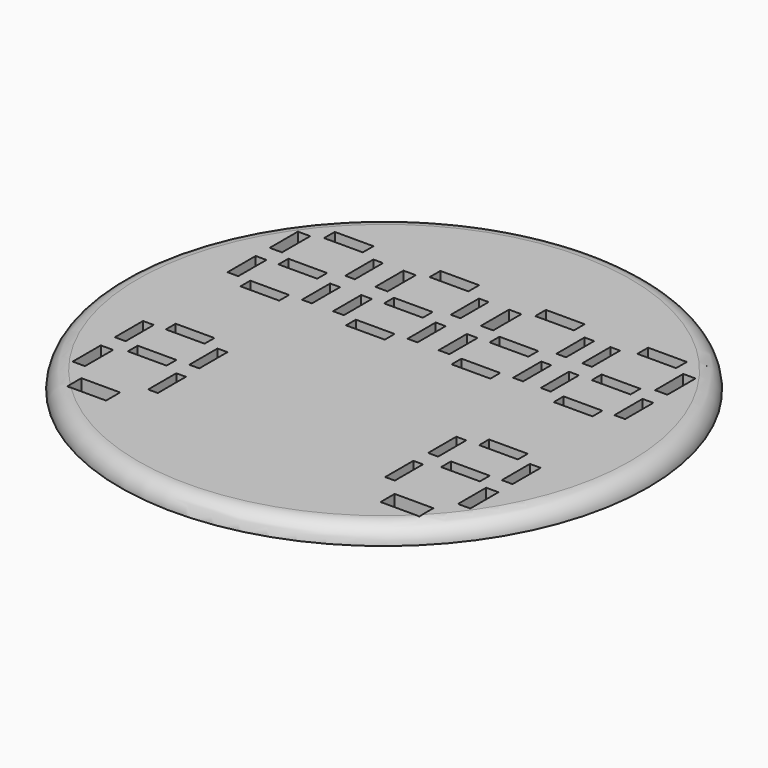
from build123d import *

# Parameters (mm, degrees)
F0_R     = 15
F0_W     = 2.201593481
F0_H     = 1
F0_W_2   = 0.7
F0_H_2   = 2
F0_W_3   = 0.611269173
F0_H_3   = 0.7
F0_W_4   = 0.547691976
F0_W_5   = 0.5653050612
F1_DEPTH = 1


# Not quite as in the source:
# - a fillet or chamfer that OpenCascade refuses, or shapes differently, is made with other operations: its cross-section is extruded or revolved along the edge and cut away or added
# - a feature names something its author has since deleted; it is built from what else it names


with BuildPart() as f1:
    # F0 (on Top) → F1 (new body)
    with BuildSketch(Plane.XY):
        Circle(F0_R)
        with Locations((-8.9021953754, -9.5)):
            Rectangle(F0_W, F0_H, mode=Mode.SUBTRACT)
        with Locations((-10.9492010795, -7)):
            Rectangle(F0_W_2, F0_H_2, mode=Mode.SUBTRACT)
        with Locations((-10.9935664929, -4)):
            Rectangle(F0_W_3, F0_H_2, mode=Mode.SUBTRACT)
        with Locations((-8.9021953754, -5.35)):
            Rectangle(F0_W, F0_H_3, mode=Mode.SUBTRACT)
        with Locations((-8.9021953754, -2.65)):
            Rectangle(F0_W, F0_H_3, mode=Mode.SUBTRACT)
        with Locations((-6.7348206503, -7)):
            Rectangle(F0_W_4, F0_H_2, mode=Mode.SUBTRACT)
        with Locations((-6.7848820763, -4)):
            Rectangle(F0_W_5, F0_H_2, mode=Mode.SUBTRACT)
        with Locations((8.9021953754, -9.5)):
            Rectangle(F0_W, F0_H, mode=Mode.SUBTRACT)
        with Locations((6.7348206503, -7)):
            Rectangle(F0_W_4, F0_H_2, mode=Mode.SUBTRACT)
        with Locations((6.7848820763, -4)):
            Rectangle(F0_W_5, F0_H_2, mode=Mode.SUBTRACT)
        with Locations((10.9492010795, -7)):
            Rectangle(F0_W_2, F0_H_2, mode=Mode.SUBTRACT)
        with Locations((8.9021953754, -5.35)):
            Rectangle(F0_W, F0_H_3, mode=Mode.SUBTRACT)
        with Locations((10.9935664929, -4)):
            Rectangle(F0_W_3, F0_H_2, mode=Mode.SUBTRACT)
        with Locations((8.9021953754, -2.65)):
            Rectangle(F0_W, F0_H_3, mode=Mode.SUBTRACT)
        with Locations((-8.9021953754, 2.65)):
            Rectangle(F0_W, F0_H_3, mode=Mode.SUBTRACT)
        with Locations((-10.9935664929, 4)):
            Rectangle(F0_W_3, F0_H_2, mode=Mode.SUBTRACT)
        with Locations((-8.9021953754, 5.35)):
            Rectangle(F0_W, F0_H_3, mode=Mode.SUBTRACT)
        with Locations((-10.9492010795, 7)):
            Rectangle(F0_W_2, F0_H_2, mode=Mode.SUBTRACT)
        with Locations((-2.9021953754, 2.65)):
            Rectangle(F0_W, F0_H_3, mode=Mode.SUBTRACT)
        with Locations((-6.7848820763, 4)):
            Rectangle(F0_W_5, F0_H_2, mode=Mode.SUBTRACT)
        with Locations((-4.9935664929, 4)):
            Rectangle(F0_W_3, F0_H_2, mode=Mode.SUBTRACT)
        with Locations((-6.7348206503, 7)):
            Rectangle(F0_W_4, F0_H_2, mode=Mode.SUBTRACT)
        with Locations((-4.9492010795, 7)):
            Rectangle(F0_W_2, F0_H_2, mode=Mode.SUBTRACT)
        with Locations((-2.9021953754, 5.35)):
            Rectangle(F0_W, F0_H_3, mode=Mode.SUBTRACT)
        with Locations((-0.7848820763, 4)):
            Rectangle(F0_W_5, F0_H_2, mode=Mode.SUBTRACT)
        with Locations((-0.7348206503, 7)):
            Rectangle(F0_W_4, F0_H_2, mode=Mode.SUBTRACT)
        Polygon((-10.0029921159, 9), (-7.8013986349, 9), (-7.8024366548, 8.2387067378), (-10.0029921159, 8.2387067378), align=None, mode=Mode.SUBTRACT)
        Polygon((-1.8024366548, 8.2387067378), (-4.0029921159, 8.2387067378), (-4.0029921159, 9), (-1.8013986349, 9), align=None, mode=Mode.SUBTRACT)
        with Locations((3.0978046246, 2.65)):
            Rectangle(F0_W, F0_H_3, mode=Mode.SUBTRACT)
        with Locations((1.0064335071, 4)):
            Rectangle(F0_W_3, F0_H_2, mode=Mode.SUBTRACT)
        with Locations((3.0978046246, 5.35)):
            Rectangle(F0_W, F0_H_3, mode=Mode.SUBTRACT)
        with Locations((1.0507989205, 7)):
            Rectangle(F0_W_2, F0_H_2, mode=Mode.SUBTRACT)
        with Locations((5.2151179237, 4)):
            Rectangle(F0_W_5, F0_H_2, mode=Mode.SUBTRACT)
        with Locations((6.7848820763, 4)):
            Rectangle(F0_W_5, F0_H_2, mode=Mode.SUBTRACT)
        with Locations((5.2651793497, 7)):
            Rectangle(F0_W_4, F0_H_2, mode=Mode.SUBTRACT)
        with Locations((6.7348206503, 7)):
            Rectangle(F0_W_4, F0_H_2, mode=Mode.SUBTRACT)
        with Locations((8.9021953754, 2.65)):
            Rectangle(F0_W, F0_H_3, mode=Mode.SUBTRACT)
        with Locations((8.9021953754, 5.35)):
            Rectangle(F0_W, F0_H_3, mode=Mode.SUBTRACT)
        with Locations((10.9935664929, 4)):
            Rectangle(F0_W_3, F0_H_2, mode=Mode.SUBTRACT)
        with Locations((10.9492010795, 7)):
            Rectangle(F0_W_2, F0_H_2, mode=Mode.SUBTRACT)
        Polygon((4.1975633452, 8.2387067378), (1.9970078841, 8.2387067378), (1.9970078841, 9), (4.1986013651, 9), align=None, mode=Mode.SUBTRACT)
        Polygon((10.0029921159, 9), (10.0029921159, 8.2387067378), (7.8024366548, 8.2387067378), (7.8013986349, 9), align=None, mode=Mode.SUBTRACT)
    extrude(amount=F1_DEPTH)

    # F2: fillet of radius 1 on 1 edges, made by hand

    # F2_s1 → F2_t2 (revolve, cut)
    with BuildSketch(Plane.XZ):
        with BuildLine():
            ThreePointArc((15, 0), (14.7071067812, 0.7071067812), (14, 1))
            Line((14, 1), (15, 1))
            Line((15, 1), (15, 0))
        make_face()
    revolve(axis=Axis((0, 0, 1), (0, 0, 1)), mode=Mode.SUBTRACT)


solid = f1.part
